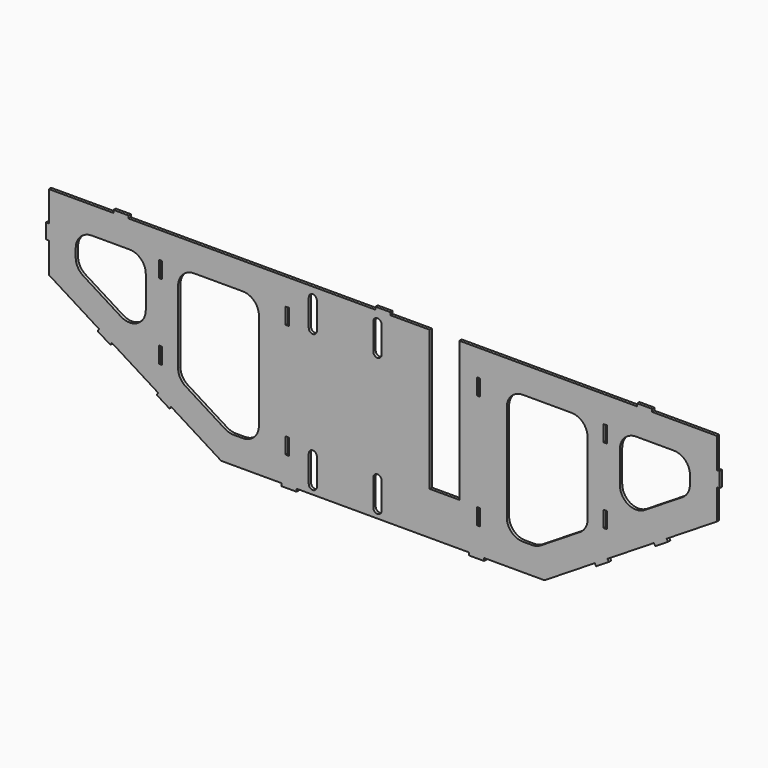
from build123d import *

# Parameters (mm, degrees)
F0_W     = 3.81
F0_H     = 19.05
F1_DEPTH = 3.429


# Not quite as in the source:
# - ends of sketch curves that miss each other by under 0.0002 mm in the source are joined


with BuildPart() as f1:
    # F0 (on Front) → F1 (new body)
    with BuildSketch(Plane.XZ):
        Polygon((65.6458174, -303.6329462), (62.4708174, -303.6329462), (62.4708174, -321.4129462), (65.6458174, -321.4129462), (65.6458174, -356.9729462), (124.8784904, -393.99337), (123.1957404, -396.68577), (138.273155, -406.1091446), (139.955905, -403.4167446), (194.5357298, -437.5291224), (192.8529798, -440.2215224), (207.9303944, -449.644897), (209.6131444, -446.9525224), (268.8458174, -483.9729462), (339.9658174, -483.9729462), (339.9658174, -487.1479462), (357.7458174, -487.1479462), (357.7458174, -483.9729462), (560.9458174, -483.9729462), (560.9458174, -487.1479462), (578.7258174, -487.1479462), (578.7258174, -483.9729462), (649.8458174, -483.9729462), (709.0784904, -446.9525224), (710.7612404, -449.644897), (725.838655, -440.2215224), (724.155905, -437.5291224), (778.7357298, -403.4167446), (780.4184798, -406.1091446), (795.495869, -396.68577), (793.8131444, -393.99337), (853.0458174, -356.9729462), (853.0458174, -321.4129462), (856.2208174, -321.4129462), (856.2208174, -303.6329462), (853.0458174, -303.6329462), (853.0458174, -268.0729462), (776.8458174, -268.0729462), (776.8458174, -264.8979462), (759.0658174, -264.8979462), (759.0658174, -268.0729462), (549.5158174, -268.0729462), (549.5158174, -433.1729462), (514.5908174, -433.1729462), (514.5908174, -268.0729462), (468.2358174, -268.0729462), (468.2358174, -264.8979462), (450.4558174, -264.8979462), (450.4558174, -268.0729462), (159.6258174, -268.0729462), (159.6258174, -264.8979462), (141.8458174, -264.8979462), (141.8458174, -268.0729462), (65.6458174, -268.0729462), align=None)
        with Locations((346.6968174, -443.3329462)):
            Rectangle(F0_W, F0_H, mode=Mode.SUBTRACT)
        with BuildLine():
            ThreePointArc((372.0333174, -442.6979462), (376.7958174, -437.9354462), (381.5583174, -442.6979462))
            Line((381.5583174, -442.6979462), (381.5583174, -474.4479462))
            ThreePointArc((381.5583174, -474.4479462), (376.7958174, -479.2104462), (372.0333174, -474.4479462))
            Line((372.0333174, -474.4479462), (372.0333174, -442.6979462))
        make_face(mode=Mode.SUBTRACT)
        with BuildLine():
            ThreePointArc((457.7583174, -474.4479462), (452.9958174, -479.2104462), (448.2333174, -474.4479462))
            Line((448.2333174, -474.4479462), (448.2333174, -442.6979462))
            ThreePointArc((448.2333174, -442.6979462), (452.9958174, -437.9354462), (457.7583174, -442.6979462))
            Line((457.7583174, -442.6979462), (457.7583174, -474.4479462))
        make_face(mode=Mode.SUBTRACT)
        with Locations((197.3448174, -397.6129462)):
            Rectangle(F0_W, F0_H, mode=Mode.SUBTRACT)
        with Locations((571.9948174, -443.3329462)):
            Rectangle(F0_W, F0_H, mode=Mode.SUBTRACT)
        with Locations((721.3468174, -397.6129462)):
            Rectangle(F0_W, F0_H, mode=Mode.SUBTRACT)
        with BuildLine():
            ThreePointArc((179.9458174, -356.5983978), (170.1306614744, -373.26033511), (150.7993444424, -372.7527697722))
            Line((150.7993444424, -372.7527697722), (106.3493428, -344.9715224))
            ThreePointArc((106.3493428, -344.9715224), (99.78388009, -338.0519918744), (97.3958174, -328.8171478))
            Line((97.3958174, -328.8171478), (97.3958174, -318.8729462))
            ThreePointArc((97.3958174, -318.8729462), (102.9754332184, -305.4025620184), (116.4458174, -299.8229462))
            Line((116.4458174, -299.8229462), (160.8958174, -299.8229462))
            ThreePointArc((160.8958174, -299.8229462), (174.3662015816, -305.4025620184), (179.9458174, -318.8729462))
            Line((179.9458174, -318.8729462), (179.9458174, -356.5983978))
        make_face(mode=Mode.SUBTRACT)
        with BuildLine():
            ThreePointArc((226.9993444424, -420.3777697722), (220.43388009, -413.4582418744), (218.0458174, -404.2233978))
            Line((218.0458174, -404.2233978), (218.0458174, -318.8729462))
            ThreePointArc((218.0458174, -318.8729462), (223.6254332184, -305.4025620184), (237.0958174, -299.8229462))
            Line((237.0958174, -299.8229462), (294.2458174, -299.8229462))
            ThreePointArc((294.2458174, -299.8229462), (307.7162015816, -305.4025620184), (313.2958174, -318.8729462))
            Line((313.2958174, -318.8729462), (313.2958174, -433.1729462))
            ThreePointArc((313.2958174, -433.1729462), (307.7162015816, -446.6433303816), (294.2458174, -452.2229462))
            Line((294.2458174, -452.2229462), (283.4150542, -452.2229462))
            ThreePointArc((283.4150542, -452.2229462), (278.1632997385, -451.4847340722), (273.3185698266, -449.3273110374))
            Line((273.3185698266, -449.3273110374), (226.9993444424, -420.3777697722))
        make_face(mode=Mode.SUBTRACT)
        with Locations((197.3448174, -308.7129462)):
            Rectangle(F0_W, F0_H, mode=Mode.SUBTRACT)
        with Locations((346.6968174, -308.7129462)):
            Rectangle(F0_W, F0_H, mode=Mode.SUBTRACT)
        with BuildLine():
            ThreePointArc((372.0333174, -280.7729462), (376.7958174, -276.0104462), (381.5583174, -280.7729462))
            Line((381.5583174, -280.7729462), (381.5583174, -312.5229462))
            ThreePointArc((381.5583174, -312.5229462), (376.7958174, -317.2854462), (372.0333174, -312.5229462))
            Line((372.0333174, -312.5229462), (372.0333174, -280.7729462))
        make_face(mode=Mode.SUBTRACT)
        with BuildLine():
            ThreePointArc((457.7583174, -312.5229462), (452.9958174, -317.2854462), (448.2333174, -312.5229462))
            Line((448.2333174, -312.5229462), (448.2333174, -280.7729462))
            ThreePointArc((448.2333174, -280.7729462), (452.9958174, -276.0104462), (457.7583174, -280.7729462))
            Line((457.7583174, -280.7729462), (457.7583174, -312.5229462))
        make_face(mode=Mode.SUBTRACT)
        with BuildLine():
            ThreePointArc((624.4458174, -452.2229462), (610.9754332184, -446.6433303816), (605.3958174, -433.1729462))
            Line((605.3958174, -433.1729462), (605.3958174, -318.8729462))
            ThreePointArc((605.3958174, -318.8729462), (610.9754332184, -305.4025620184), (624.4458174, -299.8229462))
            Line((624.4458174, -299.8229462), (681.5958174, -299.8229462))
            ThreePointArc((681.5958174, -299.8229462), (695.0662015816, -305.4025620184), (700.6458174, -318.8729462))
            Line((700.6458174, -318.8729462), (700.6458174, -404.2233978))
            ThreePointArc((700.6458174, -404.2233978), (698.25775471, -413.4582418744), (691.6922903576, -420.3777697722))
            Line((691.6922903576, -420.3777697722), (645.3730552, -449.3272954))
            ThreePointArc((645.3730552, -449.3272954), (640.5283200138, -451.4847311032), (635.2765552, -452.2229462))
            Line((635.2765552, -452.2229462), (624.4458174, -452.2229462))
        make_face(mode=Mode.SUBTRACT)
        with BuildLine():
            ThreePointArc((738.7458174, -318.8729462), (744.3254332184, -305.4025620184), (757.7958174, -299.8229462))
            Line((757.7958174, -299.8229462), (802.2458174, -299.8229462))
            ThreePointArc((802.2458174, -299.8229462), (815.7162015816, -305.4025620184), (821.2958174, -318.8729462))
            Line((821.2958174, -318.8729462), (821.2958174, -328.8171478))
            ThreePointArc((821.2958174, -328.8171478), (818.90775471, -338.0519918744), (812.3422903576, -344.9715197722))
            Line((812.3422903576, -344.9715197722), (767.892292, -372.7527724))
            ThreePointArc((767.892292, -372.7527724), (748.5609733256, -373.26033511), (738.7458174, -356.5983978))
            Line((738.7458174, -356.5983978), (738.7458174, -318.8729462))
        make_face(mode=Mode.SUBTRACT)
        with Locations((571.9948174, -308.7129462)):
            Rectangle(F0_W, F0_H, mode=Mode.SUBTRACT)
        with Locations((721.3468174, -308.7129462)):
            Rectangle(F0_W, F0_H, mode=Mode.SUBTRACT)
    extrude(amount=F1_DEPTH)


solid = f1.part
